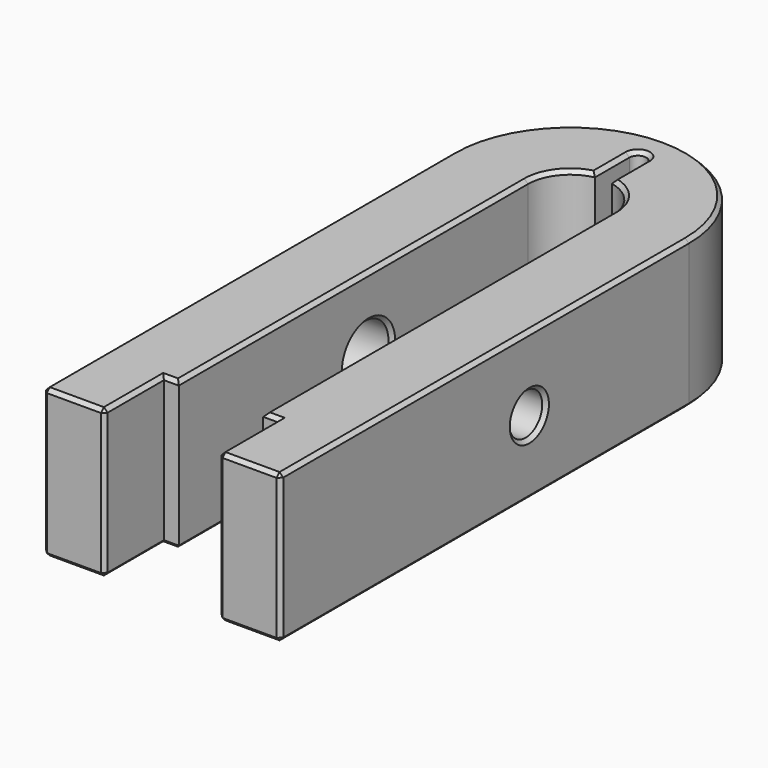
from build123d import *

# Parameters (mm, degrees)
F1_DEPTH       = 10
F3_D           = 2.8
F3_CBORE_D     = 4
F3_CBORE_DEPTH = 6
F4_SIZE        = 0.25


with BuildPart() as f1:
    # F0 (on Top) → F1 (new body)
    with BuildSketch(Plane.XY):
        with BuildLine():
            Line((3.85, -20), (8, -20))
            Line((8, -20), (8, 14.4496737048))
            ThreePointArc((8, 14.4496737048), (0, 22.4496737048), (-8, 14.4496737048))
            Line((-8, 14.4496737048), (-8, -20))
            Line((-8, -20), (-3.85, -20))
            Line((-3.85, -20), (-3.85, -15))
            Line((-3.85, -15), (-2.85, -15))
            Line((-2.85, -15), (-2.85, 14.4496737048))
            ThreePointArc((-2.85, 14.4496737048), (-2.2074806008, 16.252318816), (-0.5696284934, 17.2421678193))
            Line((-0.5696284934, 17.2421678193), (-0.5696284934, 20.1496737048))
            ThreePointArc((-0.5696284934, 20.1496737048), (0, 20.7193021982), (0.5696284934, 20.1496737048))
            Line((0.5696284934, 20.1496737048), (0.5696284934, 17.2421678193))
            ThreePointArc((0.5696284934, 17.2421678193), (2.2074806008, 16.252318816), (2.85, 14.4496737048))
            Line((2.85, 14.4496737048), (2.85, -15))
            Line((2.85, -15), (3.85, -15))
            Line((3.85, -15), (3.85, -20))
        make_face()
    extrude(amount=F1_DEPTH)

    # F3 (through all)
    with Locations(Plane(origin=(-8, 0, 0), x_dir=(0, -1, 0), z_dir=(-1, 0, 0))):
        with Locations((-1, 5)):
            CounterBoreHole(F3_D / 2, F3_CBORE_D / 2, F3_CBORE_DEPTH)

    # F4
    f4_edges = [f1.edges().sort_by_distance(p)[0] for p in [
        (5.925, -20, 0),
        (8, -2.775163, 0),
        (0, 22.449674, 0),
        (-8, -2.775163, 0),
        (-5.925, -20, 0),
        (-3.85, -17.5, 0),
        (-3.35, -15, 0),
        (-2.85, -0.275163, 0),
        (-2.207481, 16.252319, 0),
        (-0.569628, 18.695921, 0),
        (0, 20.719302, 0),
        (0.569628, 18.695921, 0),
        (2.207481, 16.252319, 0),
        (2.85, -0.275163, 0),
        (3.35, -15, 0),
        (3.85, -17.5, 0),
        (5.925, -20, 10),
        (8, -2.775163, 10),
        (0, 22.449674, 10),
        (-8, -2.775163, 10),
        (-5.925, -20, 10),
        (-3.85, -17.5, 10),
        (-3.35, -15, 10),
        (-2.85, -0.275163, 10),
        (-2.207481, 16.252319, 10),
        (-0.569628, 18.695921, 10),
        (0, 20.719302, 10),
        (0.569628, 18.695921, 10),
        (2.207481, 16.252319, 10),
        (2.85, -0.275163, 10),
        (3.35, -15, 10),
        (3.85, -17.5, 10),
        (-8, -20, 5),
        (-3.85, -20, 5),
        (3.85, -20, 5),
        (8, -20, 5),
        (8, 2.4, 5),
        (2.85, 2.4, 5),
        (-8, 3, 5),
        (-2.85, 3, 5),
    ]]
    chamfer(f4_edges, length=F4_SIZE)


solid = f1.part
